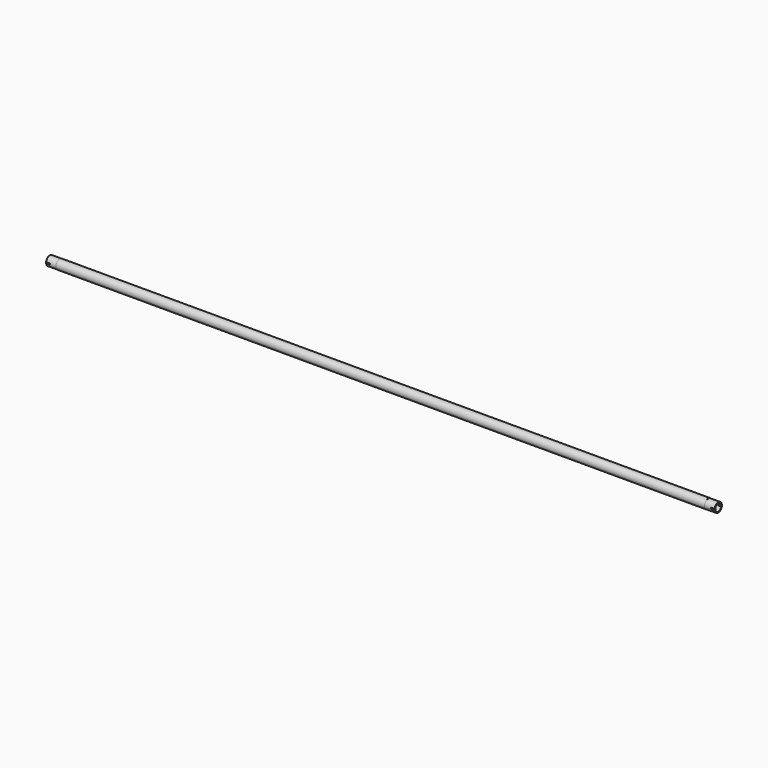
from build123d import *

# Parameters (mm, degrees)
F0_R     = 27.5
F0_R_2   = 21.5
F1_DEPTH = 1950
F2_R     = 28
F2_R_2   = 27
F3_DEPTH = 58
F5_DEPTH = 27.5


# Not quite as in the source:
# - a pattern or mirror of a feature is missing from the dataset's text; its kind, count and spacing are read off the source's solid


with BuildPart() as f1:
    # F0 (on Right) → F1 (new body, symmetric)
    with BuildSketch(Plane.YZ):
        Circle(F0_R)
        Circle(F0_R_2, mode=Mode.SUBTRACT)
    extrude(amount=F1_DEPTH, both=True)

    # F2 (on face) → F3 (cut)
    with BuildSketch(Plane.YZ.offset(1950)):
        Circle(F2_R)
        Circle(F2_R_2, mode=Mode.SUBTRACT)
    f3 = extrude(amount=-F3_DEPTH, mode=Mode.SUBTRACT)

    # F3_copies: F3 across plane
    add(f3.mirror(Plane(origin=(0, 0, 0), x_dir=(0, 0, -1), z_dir=(-1, 0, 0))), mode=Mode.SUBTRACT)

    # F4 (on Front) → F5 (cut, symmetric)
    with BuildSketch(Plane.XZ):
        with BuildLine():
            Line((-1931, 3.5), (-1940.5, 3.5))
            ThreePointArc((-1940.5, 3.5), (-1944, 0), (-1940.5, -3.5))
            Line((-1940.5, -3.5), (-1931, -3.5))
            ThreePointArc((-1931, -3.5), (-1927.5, 0), (-1931, 3.5))
        make_face()
    f5 = extrude(amount=F5_DEPTH, both=True, mode=Mode.SUBTRACT)

    # F5_copies: F5 across plane
    add(f5.mirror(Plane(origin=(0, 0, 0), x_dir=(0, 0, 1), z_dir=(1, 0, 0))), mode=Mode.SUBTRACT)


solid = f1.part
